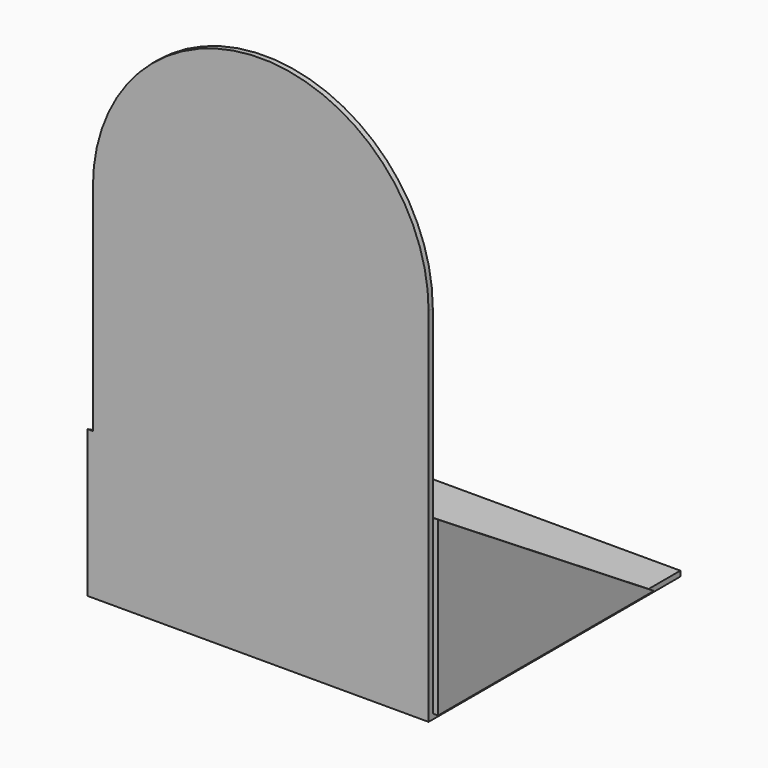
from build123d import *

# Parameters (mm, degrees)
F1_DEPTH = 6.35
F3_W     = 406.4
F3_H     = 381
F4_DEPTH = 6.35
F7_DEPTH = 6.35
F9_DEPTH = 6.35


# Not quite as in the source:
# - a feature names something its author has since deleted; it is built from what else it names


with BuildPart() as f1:
    # F0 (on Front) → F1 (new body)
    with BuildSketch(Plane.XZ):
        with BuildLine():
            Line((-203.2, 215.9), (-203.2, -215.9))
            Line((-203.2, -215.9), (203.2, -215.9))
            Line((203.2, -215.9), (203.2, 215.9))
            ThreePointArc((203.2, 215.9), (0, 419.1), (-203.2, 215.9))
        make_face()
    extrude(amount=F1_DEPTH)

    # F3 (on offset) → F4 (join)
    with BuildSketch(Plane(origin=(0, 0, -215.9), x_dir=(1, 0, 0), z_dir=(0, 0, -1))):
        with Locations((0, -184.15)):
            Rectangle(F3_W, F3_H)
    extrude(amount=F4_DEPTH)

    # F6 (on offset) → F7 (join)
    with BuildSketch(Plane(origin=(-203.2, 0, 0), x_dir=(0, -1, 0), z_dir=(-1, 0, 0))):
        Polygon((6.35, -44.45), (-336.55, -222.25), (6.35, -222.25), align=None)
    extrude(amount=F7_DEPTH)


with BuildPart() as f9:
    # F8 (on face) → F9 (new body)
    with BuildSketch(Plane.YZ.offset(203.2)):
        Polygon((0, -215.9), (326.6108695652, -215.9), (0, -7.2319444444), align=None)
    extrude(amount=F9_DEPTH)


solid = Compound([f1.part, f9.part])
